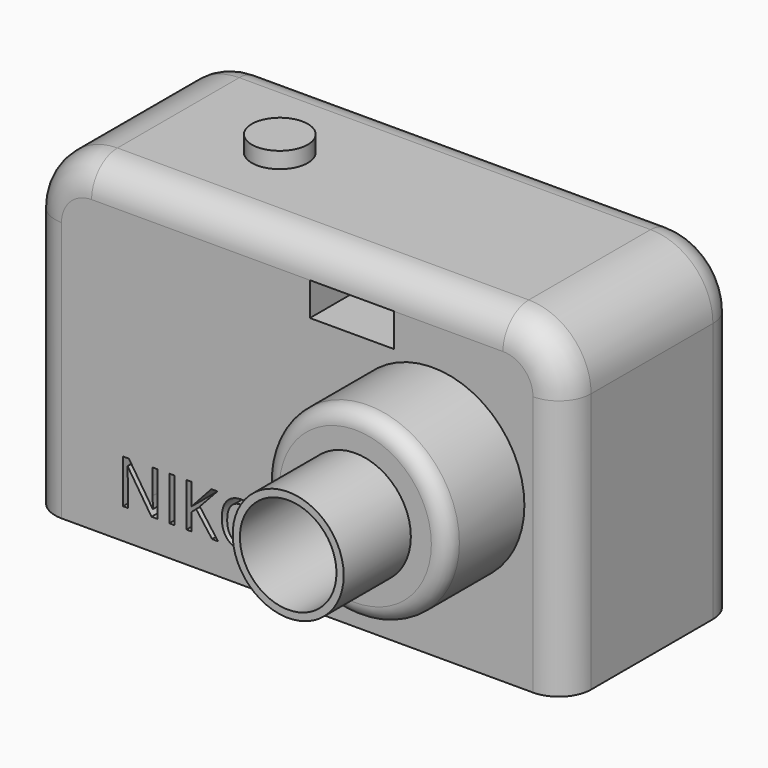
from build123d import *

# Parameters (mm, degrees)
F0_W          = 84.3707341701
F0_H          = 34.1274893872
F1_DEPTH      = 50.8
F2_R          = 14.4206092154
F3_DEPTH      = 15.24
F4_R          = 9.8113639175
F5_R          = 2.4528409794
F6_R          = 9.8113639175
F7_R          = 5.08
F8_TEXT_SIZE  = 10.8001559538
F9_DEPTH      = 19.304
F10_TEXT_SIZE = 13.1664684482
F11_DEPTH     = 20.574
F12_TEXT_SIZE = 9.6511412671
F13_DEPTH     = 11.43
F14_R         = 8.7399968066
F15_DEPTH     = 13.208
F16_R         = 7.5999151257
F17_DEPTH     = 28.702
F18_R         = 4.4109369962
F19_DEPTH     = 2.54
F20_W         = 13.2718025707
F20_H         = 5.2410067928
F21_DEPTH     = 17.018
F22_TEXT_SIZE = 8.3443875198
F23_DEPTH     = 9.144
F24_W         = 10.2718663402
F24_H         = 5.2645802498
F25_DEPTH     = 10.922
F27_DEPTH     = 5.334


# Not quite as in the source:
# - Text() gives the source's letters only with a copy of the font that has no kerning and outlines rounded to 1/6400 em; it was checked with that copy


with BuildPart() as f1:
    # F0 (on Top) → F1 (new body)
    with BuildSketch(Plane.XY):
        with Locations((0.9479885921, 0.4739932265)):
            Rectangle(F0_W, F0_H)
    extrude(amount=F1_DEPTH)

    # F2 (on face) → F3 (join)
    with BuildSketch(Plane.XZ.offset(16.5897514671)):
        with Locations((22.2776662558, 25.5008172244)):
            Circle(F2_R)
    extrude(amount=F3_DEPTH)

    # F4
    f4_edges = [f1.edges().sort_by_distance(p)[0] for p in [
        (-41.237378, 0.473993, 50.8),
    ]]
    fillet(f4_edges, radius=F4_R)

    # F5
    f5_edges = [f1.edges().sort_by_distance(p)[0] for p in [
        (7.857057, -31.829751, 25.500817),
    ]]
    fillet(f5_edges, radius=F5_R)

    # F6
    f6_edges = [f1.edges().sort_by_distance(p)[0] for p in [
        (43.133356, 0.473993, 50.8),
    ]]
    fillet(f6_edges, radius=F6_R)

    # F7
    f7_edges = [f1.edges().sort_by_distance(p)[0] for p in [
        (0.947989, -16.589751, 50.8),
        (0.947989, 17.537738, 50.8),
    ]]
    fillet(f7_edges, radius=F7_R)

    # F8 (on face) → F9 (join)
    with BuildSketch(Plane.XZ.offset(16.5897514671)):
        with Locations((-33.9749280965, 4.2018611014)):
            Text('NIKON', F8_TEXT_SIZE, font='Open Sans', text_align=(TextAlign.LEFT, TextAlign.BOTTOM))
    extrude(amount=-F9_DEPTH)

    # F10 (on face) → F11 (join)
    with BuildSketch(Plane.XZ.offset(16.5897514671)):
        with Locations((-33.2743003964, 2.749158768)):
            Text('Camera', F10_TEXT_SIZE, font='Open Sans', text_align=(TextAlign.LEFT, TextAlign.BOTTOM))
    extrude(amount=-F11_DEPTH)

    # F12 (on face) → F13 (cut)
    with BuildSketch(Plane.XZ.offset(16.5897514671)):
        with Locations((-27.4104699492, 4.8365169205)):
            Text('NIKON', F12_TEXT_SIZE, font='Open Sans', text_align=(TextAlign.LEFT, TextAlign.BOTTOM))
    extrude(amount=-F13_DEPTH, mode=Mode.SUBTRACT)

    # F14 (on face) → F15 (join)
    with BuildSketch(Plane.XZ.offset(31.8297514671)):
        with Locations((22.2776662558, 25.5008172244)):
            Circle(F14_R)
    extrude(amount=F15_DEPTH)

    # F16 (on face) → F17 (cut)
    with BuildSketch(Plane.XZ.offset(45.0377514671)):
        with Locations((22.2776662558, 25.5008172244)):
            Circle(F16_R)
    extrude(amount=-F17_DEPTH, mode=Mode.SUBTRACT)

    # F18 (on face) → F19 (join)
    with BuildSketch(Plane.XY.offset(50.8)):
        with Locations((-15.0729743764, 0)):
            Circle(F18_R)
    extrude(amount=F19_DEPTH)

    # F20 (on face) → F21 (cut)
    with BuildSketch(Plane.XZ.offset(16.5897514671)):
        with Locations((9.5746566076, 43.0994966036)):
            Rectangle(F20_W, F20_H)
    extrude(amount=-F21_DEPTH, mode=Mode.SUBTRACT)

    # F22 (on face) → F23 (cut)
    with BuildSketch(Plane(origin=(0, 17.5377379201, 0), x_dir=(-1, 0, 0), z_dir=(0, 1, 0))):
        with Locations((-33.3219917596, 34.9806770682)):
            Text('HD', F22_TEXT_SIZE, font='Open Sans', text_align=(TextAlign.LEFT, TextAlign.BOTTOM))
    extrude(amount=-F23_DEPTH, mode=Mode.SUBTRACT)

    # F24 (on face) → F25 (cut)
    with BuildSketch(Plane(origin=(0, 17.5377379201, 0), x_dir=(-1, 0, 0), z_dir=(0, 1, 0))):
        with Locations((-12.826498365, 37.9583612084)):
            Rectangle(F24_W, F24_H)
    extrude(amount=-F25_DEPTH, mode=Mode.SUBTRACT)

    # F26 (on face) → F27 (cut)
    with BuildSketch(Plane(origin=(0, 17.5377379201, 0), x_dir=(-1, 0, 0), z_dir=(0, 1, 0))):
        with BuildLine():
            add(Edge.make_bspline(
                [(7.6786852442, 36.3078564405), (9.1575399845, 40.6654249971), (34.4728725637, 47.5522914362), (18.2643029618, 21.8899734721), (36.9021932956, 16.315720956), (24.1232583312, -5.2027426235), (31.2782973441, 18.5115769243), (1.5230379166, 5.6810290961), (22.4925354065, 23.2688788802), (6.2946612019, 32.2297144273), (7.6786852442, 36.3078564405)],
                knots=[0, 0, 0, 0, 0.1422974422, 0.2776777017, 0.4000350319, 0.5150304089, 0.6194016147, 0.7515776607, 0.8668272983, 1, 1, 1, 1], degree=3))
        make_face()
    extrude(amount=-F27_DEPTH, mode=Mode.SUBTRACT)


solid = f1.part
